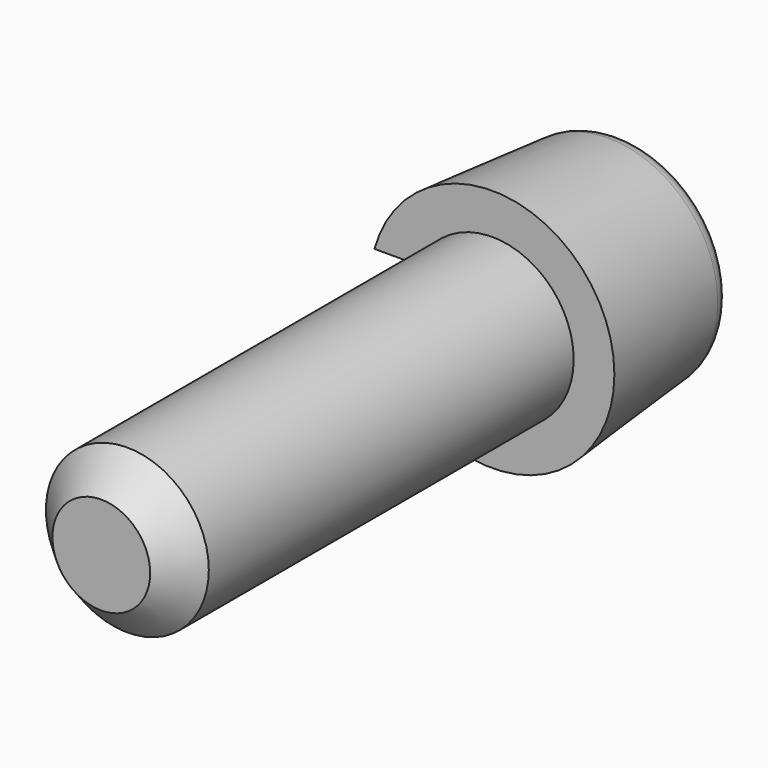
from build123d import *

# Parameters (mm, degrees)
F0_R     = 4.7625
F1_DEPTH = 6.35
F1_TAPER = 5
F2_R     = 3.175
F3_DEPTH = 19.05
F4_R     = 1.651
F5_DEPTH = 12.7
F6_SIZE  = 1.27
F7_R     = 0.762
F9_DEPTH = 4.445
F10_R    = 1.2699


# Not quite as in the source:
# - a fillet or chamfer is up to 0.001 mm smaller than in the source, because OpenCascade refuses the exact size
# - after a boolean that leaves OpenCascade's solid faulty, fix() repairs it


with BuildPart() as f1:
    # F0 (on Front) → F1 (new body)
    with BuildSketch(Plane.XZ):
        Circle(F0_R)
    extrude(amount=-F1_DEPTH, taper=F1_TAPER)

    # F2 (on face) → F3 (join)
    with BuildSketch(Plane.XZ):
        Circle(F2_R)
    extrude(amount=F3_DEPTH)

    # F4 (on face) → F5 (cut)
    with BuildSketch(Plane(origin=(0, 6.35, 0), x_dir=(-1, 0, 0), z_dir=(0, 1, 0))):
        Circle(F4_R)
    extrude(amount=-F5_DEPTH, mode=Mode.SUBTRACT)

    # F6
    f6_edges = [f1.edges().sort_by_distance(p)[0] for p in [
        (-3.175, -19.05, 0),
    ]]
    chamfer(f6_edges, length=F6_SIZE)

    # F7
    f7_edges = [f1.edges().sort_by_distance(p)[0] for p in [
        (-4.206947, 6.35, 0),
    ]]
    fillet(f7_edges, radius=F7_R)

    # F8 (on face) → F9 (cut)
    with BuildSketch(Plane.XZ):
        with BuildLine():
            ThreePointArc((-2.9099355663, -1.27), (-3.175, 0), (-2.9099355663, 1.27))
            Line((-2.9099355663, 1.27), (-4.5900442536, 1.27))
            ThreePointArc((-4.5900442536, 1.27), (-4.7625, 0), (-4.5900442536, -1.27))
            Line((-4.5900442536, -1.27), (-2.9099355663, -1.27))
        make_face()
    extrude(amount=-F9_DEPTH, mode=Mode.SUBTRACT)

    add(f1.part.fix(), mode=Mode.REPLACE)

    # F10 (radius 1.27 in the source; OpenCascade refuses exactly that, so slightly less here)
    f10_edges = [f1.edges().sort_by_distance(p)[0] for p in [
        (-3.547549, 4.445, 1.27),
        (-3.547549, 4.445, -1.27),
    ]]
    fillet(f10_edges, radius=F10_R)


solid = f1.part
